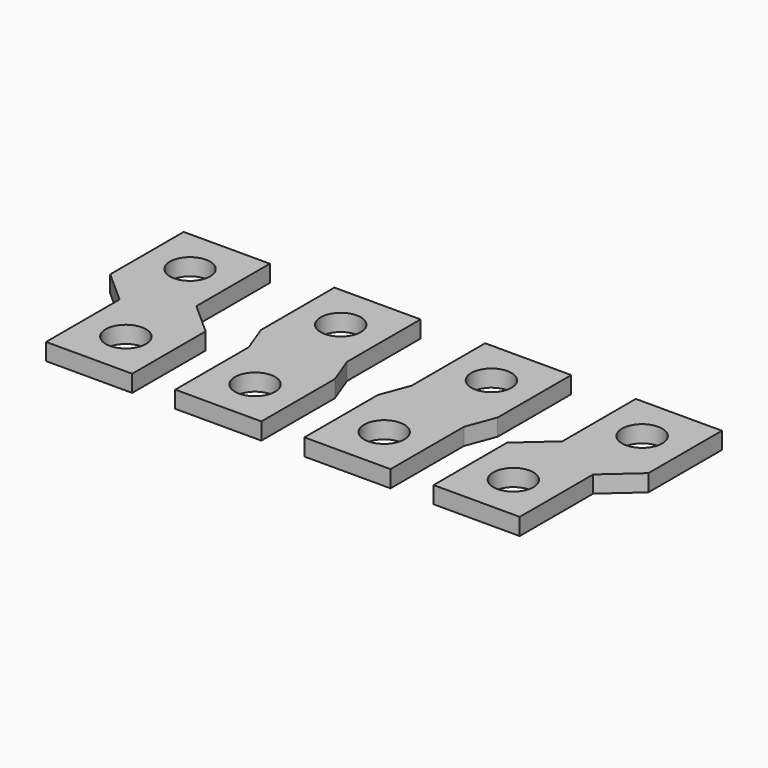
from build123d import *

# Parameters (mm, degrees)
F0_R     = 7
F1_DEPTH = 5.9


# Not quite as in the source:
# - a feature names something its author has since deleted; it is built from what else it names


with BuildPart() as f1:
    # F0 (on Top) → F1 (new body)
    with BuildSketch(Plane.XY):
        Polygon((-36.6568425298, 5), (-36.6568425298, 37), (-66.6568425298, 37), (-66.6568425298, 5), (-55.4068425298, -5), (-55.4068425298, -37), (-40.4068425298, -37), (-25.4068425298, -37), (-25.4068425298, -5), align=None)
        with BuildLine():
            ThreePointArc((-33.4068425298, -21), (-35.4570950615, -25.9497474683), (-40.4068425298, -28))
            ThreePointArc((-40.4068425298, -28), (-45.3565899981, -16.0502525317), (-33.4068425298, -21))
        make_face(mode=Mode.SUBTRACT)
        with Locations((-51.6568425298, 21)):
            Circle(F0_R, mode=Mode.SUBTRACT)
    extrude(amount=F1_DEPTH)


with BuildPart() as f1b:
    # F0 (on Top) → F1, piece 2 (new body)
    with BuildSketch(Plane.XY):
        Polygon((15.8431574702, 5), (15.8431574702, 37), (-14.1568425298, 37), (-14.1568425298, 5), (-10.4068425298, -5), (-10.4068425298, -37), (19.5931574702, -37), (19.5931574702, -5), align=None)
        with Locations((4.5931574702, -21)):
            Circle(F0_R, mode=Mode.SUBTRACT)
        with Locations((0.8431574702, 21)):
            Circle(F0_R, mode=Mode.SUBTRACT)
    extrude(amount=F1_DEPTH)


with BuildPart() as f1c:
    # F0 (on Top) → F1, piece 3 (new body)
    with BuildSketch(Plane.XY):
        Polygon((34.5931574702, -5), (34.5931574702, -37), (64.5931574702, -37), (64.5931574702, -5), (68.3431574702, 5), (68.3431574702, 37), (38.3431574702, 37), (38.3431574702, 5), align=None)
        with Locations((49.5931574702, -21)):
            Circle(F0_R, mode=Mode.SUBTRACT)
        with Locations((53.3431574702, 21)):
            Circle(F0_R, mode=Mode.SUBTRACT)
    extrude(amount=F1_DEPTH)


with BuildPart() as f1d:
    # F0 (on Top) → F1, piece 4 (new body)
    with BuildSketch(Plane.XY):
        Polygon((120.8431574702, 37), (90.8431574702, 37), (90.8431574702, 5), (79.5931574702, -5), (79.5931574702, -37), (94.5931574702, -37), (109.5931574702, -37), (109.5931574702, -5), (120.8431574702, 5), align=None)
        with BuildLine():
            ThreePointArc((101.5931574702, -21), (99.5429049385, -25.9497474683), (94.5931574702, -28))
            ThreePointArc((94.5931574702, -28), (89.6434100019, -16.0502525317), (101.5931574702, -21))
        make_face(mode=Mode.SUBTRACT)
        with Locations((105.8431574702, 21)):
            Circle(F0_R, mode=Mode.SUBTRACT)
    extrude(amount=F1_DEPTH)


solid = Compound([f1.part, f1b.part, f1c.part, f1d.part])
